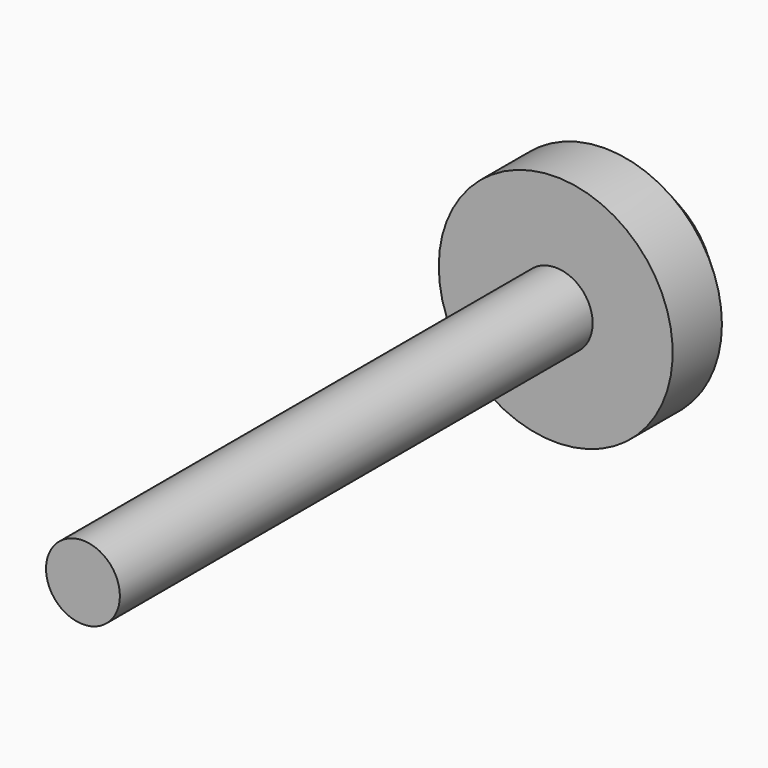
from build123d import *

# Parameters (mm, degrees)
F0_R      = 1.5
F1_DEPTH  = 12
F2_R      = 4.75
F2_R_2    = 1.5
F3_DEPTH  = 2.5
F5_R      = 3.25
F3_FACE_R = 4.75
F7_W      = 1
F7_H      = 2
F7_H_2    = 1
F7_W_2    = 2
F8_DEPTH  = 3.9
F9_R      = 0.3


with BuildPart() as f1:
    # F0 (on Front) → F1 (new body, symmetric)
    with BuildSketch(Plane.XZ):
        Circle(F0_R)
    extrude(amount=F1_DEPTH, both=True)

    # F2 (on face) → F3 (join)
    with BuildSketch(Plane(origin=(0, 12, 0), x_dir=(-1, 0, 0), z_dir=(0, 1, 0))):
        Circle(F2_R)
        Circle(F2_R_2, mode=Mode.SUBTRACT)
        Circle(F2_R_2)
    extrude(amount=F3_DEPTH)

    # F5 (on offset) → F6 section 0
    with BuildSketch(Plane.XZ.offset(-16)):
        Circle(F5_R)
    # F3_face (on face) → F6 section 1
    with BuildSketch(Plane(origin=(0, 14.5, 0), x_dir=(-1, 0, 0), z_dir=(0, 1, 0))):
        Circle(F3_FACE_R)
    loft()

    # F7 (on face) → F8 (cut)
    with BuildSketch(Plane(origin=(0, 16, 0), x_dir=(-1, 0, 0), z_dir=(0, 1, 0))):
        with Locations((0, -1.5)):
            Rectangle(F7_W, F7_H)
        Rectangle(F7_W, F7_H_2)
        with Locations((-1.5, 0)):
            Rectangle(F7_W_2, F7_H_2)
        with Locations((0, 1.5)):
            Rectangle(F7_W, F7_H)
        with Locations((1.5, 0)):
            Rectangle(F7_W_2, F7_H_2)
    extrude(amount=-F8_DEPTH, mode=Mode.SUBTRACT)

    # F9
    f9_edges = [f1.edges().sort_by_distance(p)[0] for p in [
        (-0.5, 14.05, 0.5),
        (0.5, 14.05, 0.5),
        (0.5, 14.05, -0.5),
        (-0.5, 14.05, -0.5),
    ]]
    fillet(f9_edges, radius=F9_R)


solid = f1.part
